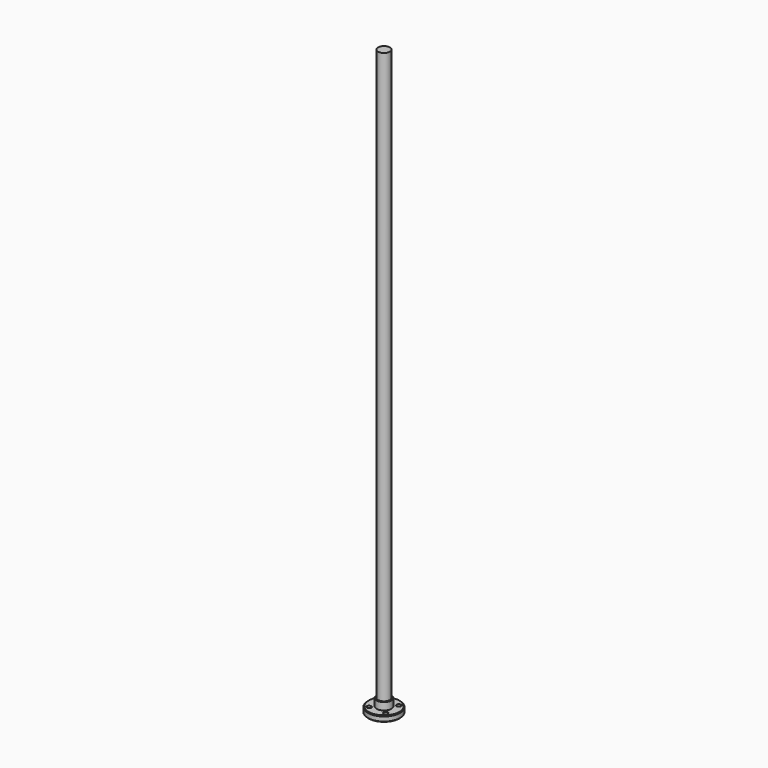
from build123d import *

# Parameters (mm, degrees)
F0_R            = 4
F1_DEPTH        = 400
F4_SIZE         = 0.5
F5_R            = 1.5
F6_DEPTH        = 25
F6_COPIES_COUNT = 4


# Not quite as in the source:
# - a pattern or mirror of a feature is missing from the dataset's text; its kind, count and spacing are read off the source's solid


with BuildPart() as f1:
    # F0 (on Top) → F1 (new body)
    with BuildSketch(Plane.XY):
        Circle(F0_R)
    extrude(amount=F1_DEPTH)


with BuildPart() as f3:
    # F2 (on Front) → F3 (revolve)
    with BuildSketch(Plane.XZ):
        Polygon((-5, 0), (-4, 0), (-4, 10), (-5, 10), (-5, 5), (-11, 5), (-11, 1), (-5, 1), align=None)
    revolve(axis=Axis((0, 0, 8.548645946), (0, 0, -1)))

    # F4
    f4_edges = [f3.edges().sort_by_distance(p)[0] for p in [
        (11, 0, 5),
        (11, 0, 1),
    ]]
    chamfer(f4_edges, length=F4_SIZE)

    # F5 (on face) → F6 (cut)
    with BuildSketch(Plane.XY.offset(5)):
        with Locations((5.6568542495, 5.6568542495)):
            Circle(F5_R)
    f6 = extrude(amount=-F6_DEPTH, mode=Mode.SUBTRACT)

    # F6_copies: F6 ×4 about axis
    f6_copies_axis = Axis((0, 0, 0), (0, 0, 1))
    for i in range(1, F6_COPIES_COUNT):
        add(f6.rotate(f6_copies_axis, i * 360 / F6_COPIES_COUNT), mode=Mode.SUBTRACT)


solid = Compound([f1.part, f3.part])
